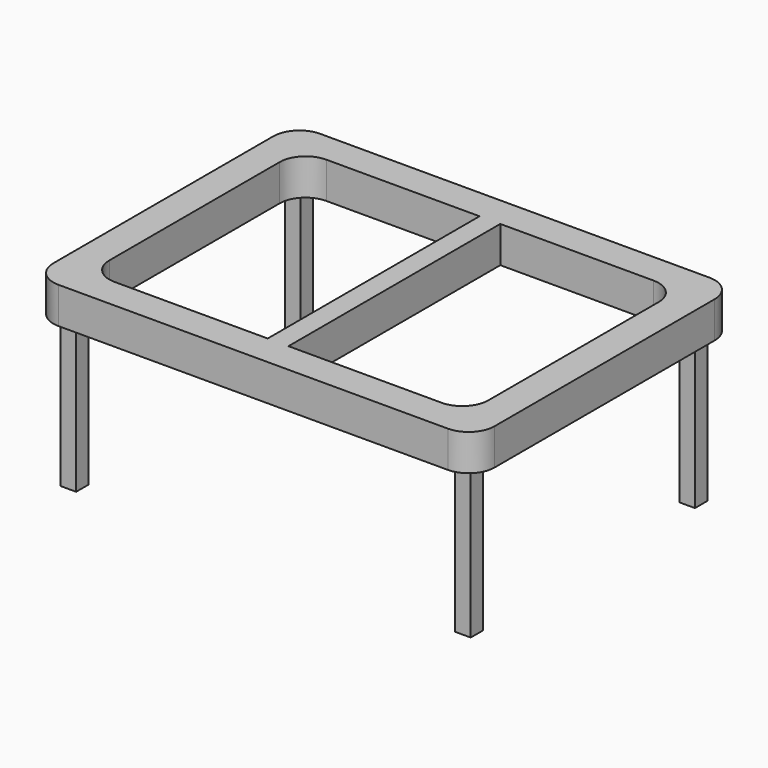
from build123d import *

# Parameters (mm, degrees)
F0_W        = 2159
F0_H        = 1600.2
F0_W_2      = 1854.2
F0_H_2      = 1295.4
F1_DEPTH    = 177.8
F2_W        = 76.2
F2_H        = 76.2
F3_DEPTH    = 736.6
F4_T1_DEPTH = 177.8
F4_T3_DEPTH = 812.8
F5_W        = 101.6
F5_H        = 177.8
F6_DEPTH    = 1295.4


# Not quite as in the source:
# - a fillet or chamfer that OpenCascade refuses, or shapes differently, is made with other operations: its cross-section is extruded or revolved along the edge and cut away or added


with BuildPart() as f1:
    # F0 (on Top) → F1 (new body)
    with BuildSketch(Plane.XY):
        with Locations((1079.5, 800.1)):
            Rectangle(F0_W, F0_H)
        with Locations((1079.5, 800.1)):
            Rectangle(F0_W_2, F0_H_2, mode=Mode.SUBTRACT)
    extrude(amount=F1_DEPTH)

    # F2 (on face) → F3 (join)
    with BuildSketch(Plane(origin=(0, 0, 0), x_dir=(1, 0, 0), z_dir=(0, 0, -1))):
        with Locations((114.3, -114.3)):
            Rectangle(F2_W, F2_H)
        with Locations((2044.7, -114.3)):
            Rectangle(F2_W, F2_H)
        with Locations((2044.7, -1485.9)):
            Rectangle(F2_W, F2_H)
        with Locations((114.3, -1485.9)):
            Rectangle(F2_W, F2_H)
    extrude(amount=F3_DEPTH)

    # F4: fillet of radius 127 on 8 edges, made by hand

    # F4_s2 → F4_t1 (join)
    with BuildSketch(Plane.XY):
        with BuildLine():
            ThreePointArc((279.4, 1447.8), (189.5974387893, 1410.6025612107), (152.4, 1320.8))
            Line((152.4, 1320.8), (152.4, 1447.8))
            Line((152.4, 1447.8), (279.4, 1447.8))
        make_face()
        with BuildLine():
            ThreePointArc((2006.6, 1320.8), (1969.4025612107, 1410.6025612107), (1879.6, 1447.8))
            Line((1879.6, 1447.8), (2006.6, 1447.8))
            Line((2006.6, 1447.8), (2006.6, 1320.8))
        make_face()
        with BuildLine():
            ThreePointArc((2006.6, 279.4), (1969.4025612107, 189.5974387893), (1879.6, 152.4))
            Line((1879.6, 152.4), (2006.6, 152.4))
            Line((2006.6, 152.4), (2006.6, 279.4))
        make_face()
        with BuildLine():
            ThreePointArc((152.4, 279.4), (189.5974387893, 189.5974387893), (279.4, 152.4))
            Line((279.4, 152.4), (152.4, 152.4))
            Line((152.4, 152.4), (152.4, 279.4))
        make_face()
    extrude(amount=F4_T1_DEPTH)

    # F4_s4 → F4_t3 (cut)
    with BuildSketch(Plane.XY.offset(-317.5)):
        with BuildLine():
            ThreePointArc((0, 127), (37.1974387893, 37.1974387893), (127, 0))
            Line((127, 0), (0, 0))
            Line((0, 0), (0, 127))
        make_face()
        with BuildLine():
            ThreePointArc((0, 1473.2), (37.1974387893, 1563.0025612107), (127, 1600.2))
            Line((127, 1600.2), (0, 1600.2))
            Line((0, 1600.2), (0, 1473.2))
        make_face()
        with BuildLine():
            ThreePointArc((2032, 0), (2121.8025612107, 37.1974387893), (2159, 127))
            Line((2159, 127), (2159, 0))
            Line((2159, 0), (2032, 0))
        make_face()
        with BuildLine():
            ThreePointArc((2032, 1600.2), (2121.8025612107, 1563.0025612107), (2159, 1473.2))
            Line((2159, 1473.2), (2159, 1600.2))
            Line((2159, 1600.2), (2032, 1600.2))
        make_face()
    extrude(amount=F4_T3_DEPTH, mode=Mode.SUBTRACT)

    # F5 (on face) → F6 (join, through all)
    with BuildSketch(Plane(origin=(0, 152.4, 0), x_dir=(-1, 0, 0), z_dir=(0, 1, 0))):
        with Locations((-1079.5, 88.9)):
            Rectangle(F5_W, F5_H)
    extrude(amount=F6_DEPTH)


solid = f1.part
